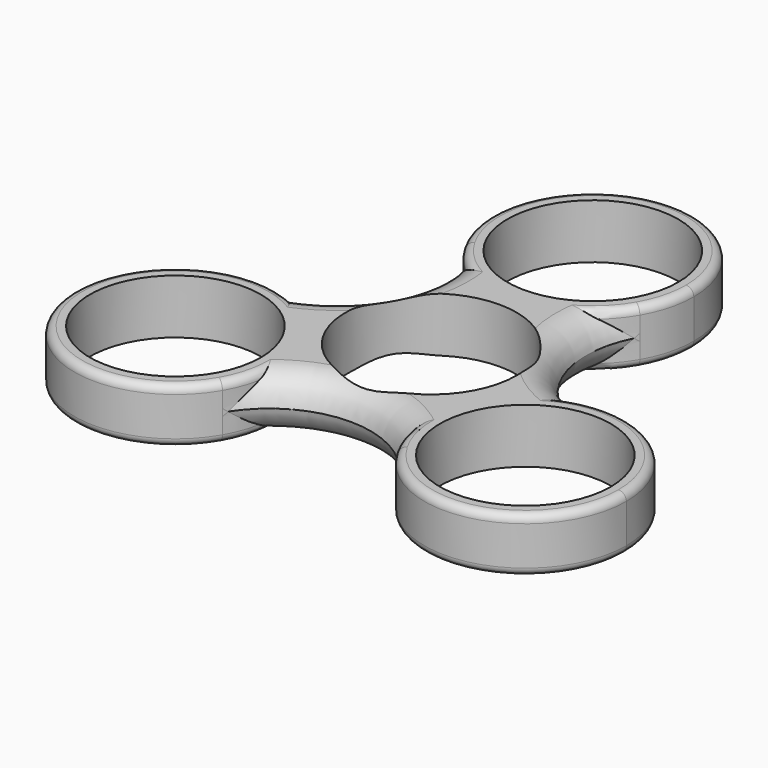
from build123d import *

# Parameters (mm, degrees)
F0_R         = 10.95
F1_DEPTH     = 7
F2_T4_ANGLE  = 119.5195556336
F2_S5_R      = 12.9500003532
F2_T6_DEPTH  = 18
F2_S7_R      = 12.9500003532
F2_T8_DEPTH  = 18
F2_T12_ANGLE = 119.5195556336
F2_S13_R     = 12.9500003532
F2_T14_DEPTH = 21
F2_S15_R     = 12.9500003532
F2_T16_DEPTH = 21
F2_T20_ANGLE = 119.5195556336
F2_S21_R     = 12.9500003532
F2_T22_DEPTH = 22
F2_S23_R     = 12.9500003532
F2_T24_DEPTH = 22
F2_T28_ANGLE = 119.5195556336
F2_S29_R     = 12.9500003532
F2_T30_DEPTH = 18
F2_S31_R     = 12.9500003532
F2_T32_DEPTH = 18
F2_T36_ANGLE = 119.5195556336
F2_S37_R     = 12.9500003532
F2_T38_DEPTH = 21
F2_S39_R     = 12.9500003532
F2_T40_DEPTH = 21
F2_T44_ANGLE = 119.5195556336
F2_S45_R     = 12.9500003532
F2_T46_DEPTH = 22
F2_S47_R     = 12.9500003532
F2_T48_DEPTH = 22
F3_R         = 1
F4_R         = 1


# Not quite as in the source:
# - a fillet or chamfer that OpenCascade refuses, or shapes differently, is made with other operations: its cross-section is extruded or revolved along the edge and cut away or added


with BuildPart() as f1:
    # F0 (on Top) → F1 (new body)
    with BuildSketch(Plane.XY):
        with BuildLine():
            ThreePointArc((-4.7e-08, 12.9500003532), (9.1570330495, 9.1570330827), (12.9500003532, 0))
            ThreePointArc((12.9500003532, 0), (12.508739778, -3.3517067761), (11.2150292324, -6.4750002674))
            ThreePointArc((11.2150292324, -6.4750002674), (15.9550583477, -1.7349710945), (22.4300585697, 0))
            ThreePointArc((22.4300585697, 0), (11.2421440333, 6.4906548839), (11.2150292849, 19.4250005297))
            ThreePointArc((11.2150292849, 19.4250005297), (6.4750001562, 14.6849714097), (-4.7e-08, 12.9500003532))
        make_face()
        with BuildLine():
            ThreePointArc((-11.2150293287, -6.4750001007), (-11.2150292747, 6.4750001942), (-4.7e-08, 12.9500003532))
            ThreePointArc((-4.7e-08, 12.9500003532), (-6.4750001969, 14.6849714332), (-11.2150292849, 19.4250005297))
            ThreePointArc((-11.2150292849, 19.4250005297), (-11.2421440333, 6.4906548839), (-22.4300585697, 0))
            ThreePointArc((-22.4300585697, 0), (-15.9550584311, -1.7349710464), (-11.2150293287, -6.4750001007))
        make_face()
        with BuildLine():
            ThreePointArc((-11.2150292849, 19.4250005297), (-6.4750001969, 14.6849714332), (-4.7e-08, 12.9500003532))
            ThreePointArc((-4.7e-08, 12.9500003532), (6.4750001562, 14.6849714097), (11.2150292849, 19.4250005297))
            ThreePointArc((11.2150292849, 19.4250005297), (12.5087397916, 22.5482939808), (12.9500003532, 25.9000007063))
            ThreePointArc((12.9500003532, 25.9000007063), (-3.3517067255, 38.4087404979), (-11.2150292849, 19.4250005297))
        make_face()
        with Locations((0, 25.9000007063)):
            Circle(F0_R, mode=Mode.SUBTRACT)
        with BuildLine():
            ThreePointArc((11.2150292849, -19.4250005297), (9.4800582165, -12.9500004056), (11.2150292324, -6.4750002674))
            ThreePointArc((11.2150292324, -6.4750002674), (-9.62e-08, -12.9500003532), (-11.2150293287, -6.4750001007))
            ThreePointArc((-11.2150293287, -6.4750001007), (-9.9213187895, -9.5982935854), (-9.4800582165, -12.9500003532))
            ThreePointArc((-9.4800582165, -12.9500003532), (-9.9213187781, -16.3017070786), (-11.2150292849, -19.4250005297))
            ThreePointArc((-11.2150292849, -19.4250005297), (0, -12.9813097678), (11.2150292849, -19.4250005297))
        make_face()
        with BuildLine():
            ThreePointArc((22.4300585697, 0), (15.9550583477, -1.7349710945), (11.2150292324, -6.4750002674))
            ThreePointArc((11.2150292324, -6.4750002674), (9.4800582165, -12.9500004056), (11.2150292849, -19.4250005297))
            ThreePointArc((11.2150292849, -19.4250005297), (25.7817652952, -25.4587401447), (35.3800589229, -12.9500003532))
            ThreePointArc((35.3800589229, -12.9500003532), (31.5870916358, -3.7929672871), (22.4300585697, 0))
        make_face()
        with Locations((22.4300585697, -12.9500003532)):
            Circle(F0_R, mode=Mode.SUBTRACT)
        with BuildLine():
            ThreePointArc((-9.4800582165, -12.9500003532), (-9.9213187895, -9.5982935854), (-11.2150293287, -6.4750001007))
            ThreePointArc((-11.2150293287, -6.4750001007), (-15.9550584311, -1.7349710464), (-22.4300585697, 0))
            ThreePointArc((-22.4300585697, 0), (-33.6450878546, -19.4250005297), (-11.2150292849, -19.4250005297))
            ThreePointArc((-11.2150292849, -19.4250005297), (-9.9213187781, -16.3017070786), (-9.4800582165, -12.9500003532))
        make_face()
        with Locations((-22.4300585697, -12.9500003532)):
            Circle(F0_R, mode=Mode.SUBTRACT)
        with BuildLine():
            ThreePointArc((11.2150292324, -6.4750002674), (12.508739778, -3.3517067761), (12.9500003532, 0))
            ThreePointArc((12.9500003532, 0), (9.1570330495, 9.1570330827), (-4.7e-08, 12.9500003532))
            ThreePointArc((-4.7e-08, 12.9500003532), (-11.2150292747, 6.4750001942), (-11.2150293287, -6.4750001007))
            ThreePointArc((-11.2150293287, -6.4750001007), (-9.62e-08, -12.9500003532), (11.2150292324, -6.4750002674))
        make_face()
        Circle(F0_R, mode=Mode.SUBTRACT)
    extrude(amount=F1_DEPTH)

    # F2: fillet of radius 4 on 6 edges, made by hand


with BuildPart() as f2_tool2:
    # F2_s3 → F2_t4 (revolve)
    with BuildSketch(Plane(origin=(-11.1333905187, 19.4716794138, 0), x_dir=(0, 0, 1), z_dir=(-0.496364659, 0.86811412, 0))):
        with BuildLine():
            ThreePointArc((2.9990343146, -0.094441514), (5.8284271247, 1.0775313612), (7.0004, 3.9069241714))
            Line((7.0004, 3.9069241714), (7.4005365685, 3.9069241714))
            ThreePointArc((7.4005365685, 3.9069241714), (7.4001365685, 1.9064413287), (7.4001365685, -0.094041514))
            Line((7.4001365685, -0.094041514), (7, -0.4941780826))
            ThreePointArc((7, -0.4941780826), (4.9995171573, -0.4941780826), (2.9990343146, -0.4945780826))
            Line((2.9990343146, -0.4945780826), (2.9990343146, -0.094441514))
        make_face()
    revolve(axis=Axis((-22.4844856895, 12.9814238654, 7), (0, 0, -1)), revolution_arc=F2_T4_ANGLE)

    # F2_s5 → F2_t6 (cut, symmetric)
    with BuildSketch(Plane.XY.offset(3.8)):
        with Locations((-22.4300585697, -12.9500003532)):
            Circle(F2_S5_R)
    extrude(amount=F2_T6_DEPTH, both=True, mode=Mode.SUBTRACT)

    # F2_s7 → F2_t8 (cut, symmetric)
    with BuildSketch(Plane.XY.offset(3.8)):
        with Locations((0, 25.9000007063)):
            Circle(F2_S7_R)
    extrude(amount=F2_T8_DEPTH, both=True, mode=Mode.SUBTRACT)


with BuildPart() as f1_1:
    add(f1.part)

    # F2_t1: cut F2_tool2
    add(f2_tool2.part, mode=Mode.SUBTRACT)


with BuildPart() as f2_tool10:
    # F2_s11 → F2_t12 (revolve)
    with BuildSketch(Plane(origin=(22.429664286, -0.0940406875, 0), x_dir=(0, 0, 1), z_dir=(0.9999912108, -0.0041926558, 0))):
        with BuildLine():
            ThreePointArc((2.9990343146, -0.094441514), (5.8284271247, 1.0775313612), (7.0004, 3.9069241714))
            Line((7.0004, 3.9069241714), (7.4005365685, 3.9069241714))
            ThreePointArc((7.4005365685, 3.9069241714), (7.4001365685, 1.9064413287), (7.4001365685, -0.094041514))
            Line((7.4001365685, -0.094041514), (7, -0.4941780826))
            ThreePointArc((7, -0.4941780826), (4.9995171573, -0.4941780826), (2.9990343146, -0.4945780826))
            Line((2.9990343146, -0.4945780826), (2.9990343146, -0.094441514))
        make_face()
    revolve(axis=Axis((22.4844856895, 12.9814238654, 7), (0, 0, -1)), revolution_arc=F2_T12_ANGLE)

    # F2_s13 → F2_t14 (cut, symmetric)
    with BuildSketch(Plane.XY.offset(5.2)):
        with Locations((22.4300585697, -12.9500003532)):
            Circle(F2_S13_R)
    extrude(amount=F2_T14_DEPTH, both=True, mode=Mode.SUBTRACT)

    # F2_s15 → F2_t16 (cut, symmetric)
    with BuildSketch(Plane.XY.offset(5.2)):
        with Locations((0, 25.9000007063)):
            Circle(F2_S15_R)
    extrude(amount=F2_T16_DEPTH, both=True, mode=Mode.SUBTRACT)


with BuildPart() as f1_2:
    add(f1_1.part)

    # F2_t9: cut F2_tool10
    add(f2_tool10.part, mode=Mode.SUBTRACT)


with BuildPart() as f2_tool18:
    # F2_s19 → F2_t20 (revolve)
    with BuildSketch(Plane(origin=(-11.2962737674, -19.3776387263, 0), x_dir=(0, 0, 1), z_dir=(-0.5036265518, -0.8639214642, 0))):
        with BuildLine():
            ThreePointArc((2.9990343146, -0.094441514), (5.8284271247, 1.0775313612), (7.0004, 3.9069241714))
            Line((7.0004, 3.9069241714), (7.4005365685, 3.9069241714))
            ThreePointArc((7.4005365685, 3.9069241714), (7.4001365685, 1.9064413287), (7.4001365685, -0.094041514))
            Line((7.4001365685, -0.094041514), (7, -0.4941780826))
            ThreePointArc((7, -0.4941780826), (4.9995171573, -0.4941780826), (2.9990343146, -0.4945780826))
            Line((2.9990343146, -0.4945780826), (2.9990343146, -0.094441514))
        make_face()
    revolve(axis=Axis((0, -25.9628477308, 7), (0, 0, -1)), revolution_arc=F2_T20_ANGLE)

    # F2_s21 → F2_t22 (cut, symmetric)
    with BuildSketch(Plane.XY.offset(3.8)):
        with Locations((-22.4300585697, -12.9500003532)):
            Circle(F2_S21_R)
    extrude(amount=F2_T22_DEPTH, both=True, mode=Mode.SUBTRACT)

    # F2_s23 → F2_t24 (cut, symmetric)
    with BuildSketch(Plane.XY.offset(3.8)):
        with Locations((22.4300585697, -12.9500003532)):
            Circle(F2_S23_R)
    extrude(amount=F2_T24_DEPTH, both=True, mode=Mode.SUBTRACT)


with BuildPart() as f1_3:
    add(f1_2.part)

    # F2_t17: cut F2_tool18
    add(f2_tool18.part, mode=Mode.SUBTRACT)


with BuildPart() as f2_tool26:
    # F2_s27 → F2_t28 (revolve)
    with BuildSketch(Plane(origin=(-11.1333905187, 19.4716794138, 0), x_dir=(0, 0, 1), z_dir=(-0.496364659, 0.86811412, 0))):
        with BuildLine():
            ThreePointArc((4.0009656854, -0.094441514), (1.1715728753, 1.0775313612), (-0.0004, 3.9069241714))
            Line((-0.0004, 3.9069241714), (-0.4005365685, 3.9069241714))
            ThreePointArc((-0.4005365685, 3.9069241714), (-0.4001365685, 1.9064413287), (-0.4001365685, -0.094041514))
            Line((-0.4001365685, -0.094041514), (0, -0.4941780826))
            ThreePointArc((0, -0.4941780826), (2.0004828427, -0.4941780826), (4.0009656854, -0.4945780826))
            Line((4.0009656854, -0.4945780826), (4.0009656854, -0.094441514))
        make_face()
    revolve(axis=Axis((-22.4844856895, 12.9814238654, 0), (0, 0, -1)), revolution_arc=F2_T28_ANGLE)

    # F2_s29 → F2_t30 (cut, symmetric)
    with BuildSketch(Plane.XY.offset(3.2)):
        with Locations((-22.4300585697, -12.9500003532)):
            Circle(F2_S29_R)
    extrude(amount=F2_T30_DEPTH, both=True, mode=Mode.SUBTRACT)

    # F2_s31 → F2_t32 (cut, symmetric)
    with BuildSketch(Plane.XY.offset(3.2)):
        with Locations((0, 25.9000007063)):
            Circle(F2_S31_R)
    extrude(amount=F2_T32_DEPTH, both=True, mode=Mode.SUBTRACT)


with BuildPart() as f1_4:
    add(f1_3.part)

    # F2_t25: cut F2_tool26
    add(f2_tool26.part, mode=Mode.SUBTRACT)


with BuildPart() as f2_tool34:
    # F2_s35 → F2_t36 (revolve)
    with BuildSketch(Plane(origin=(22.429664286, -0.0940406875, 0), x_dir=(0, 0, 1), z_dir=(0.9999912108, -0.0041926558, 0))):
        with BuildLine():
            ThreePointArc((4.0009656854, -0.094441514), (1.1715728753, 1.0775313612), (-0.0004, 3.9069241714))
            Line((-0.0004, 3.9069241714), (-0.4005365685, 3.9069241714))
            ThreePointArc((-0.4005365685, 3.9069241714), (-0.4001365685, 1.9064413287), (-0.4001365685, -0.094041514))
            Line((-0.4001365685, -0.094041514), (0, -0.4941780826))
            ThreePointArc((0, -0.4941780826), (2.0004828427, -0.4941780826), (4.0009656854, -0.4945780826))
            Line((4.0009656854, -0.4945780826), (4.0009656854, -0.094441514))
        make_face()
    revolve(axis=Axis((22.4844856895, 12.9814238654, 0), (0, 0, -1)), revolution_arc=F2_T36_ANGLE)

    # F2_s37 → F2_t38 (cut, symmetric)
    with BuildSketch(Plane.XY.offset(1.8)):
        with Locations((22.4300585697, -12.9500003532)):
            Circle(F2_S37_R)
    extrude(amount=F2_T38_DEPTH, both=True, mode=Mode.SUBTRACT)

    # F2_s39 → F2_t40 (cut, symmetric)
    with BuildSketch(Plane.XY.offset(1.8)):
        with Locations((0, 25.9000007063)):
            Circle(F2_S39_R)
    extrude(amount=F2_T40_DEPTH, both=True, mode=Mode.SUBTRACT)


with BuildPart() as f1_5:
    add(f1_4.part)

    # F2_t33: cut F2_tool34
    add(f2_tool34.part, mode=Mode.SUBTRACT)


with BuildPart() as f2_tool42:
    # F2_s43 → F2_t44 (revolve)
    with BuildSketch(Plane(origin=(-11.2962737674, -19.3776387263, 0), x_dir=(0, 0, 1), z_dir=(-0.5036265518, -0.8639214642, 0))):
        with BuildLine():
            ThreePointArc((4.0009656854, -0.094441514), (1.1715728753, 1.0775313612), (-0.0004, 3.9069241714))
            Line((-0.0004, 3.9069241714), (-0.4005365685, 3.9069241714))
            ThreePointArc((-0.4005365685, 3.9069241714), (-0.4001365685, 1.9064413287), (-0.4001365685, -0.094041514))
            Line((-0.4001365685, -0.094041514), (0, -0.4941780826))
            ThreePointArc((0, -0.4941780826), (2.0004828427, -0.4941780826), (4.0009656854, -0.4945780826))
            Line((4.0009656854, -0.4945780826), (4.0009656854, -0.094441514))
        make_face()
    revolve(axis=Axis((0, -25.9628477308, 0), (0, 0, -1)), revolution_arc=F2_T44_ANGLE)

    # F2_s45 → F2_t46 (cut, symmetric)
    with BuildSketch(Plane.XY.offset(3.2)):
        with Locations((-22.4300585697, -12.9500003532)):
            Circle(F2_S45_R)
    extrude(amount=F2_T46_DEPTH, both=True, mode=Mode.SUBTRACT)

    # F2_s47 → F2_t48 (cut, symmetric)
    with BuildSketch(Plane.XY.offset(3.2)):
        with Locations((22.4300585697, -12.9500003532)):
            Circle(F2_S47_R)
    extrude(amount=F2_T48_DEPTH, both=True, mode=Mode.SUBTRACT)


with BuildPart() as f1_6:
    add(f1_5.part)

    # F2_t41: cut F2_tool42
    add(f2_tool42.part, mode=Mode.SUBTRACT)

    # F3
    f3_edges = [f1_6.edges().sort_by_distance(p)[0] for p in [
        (0, 38.850001, 7),
        (9.80296, -15.823828, 7),
        (-33.645088, -19.425001, 7),
    ]]
    fillet(f3_edges, radius=F3_R)

    # F4
    f4_edges = [f1_6.edges().sort_by_distance(p)[0] for p in [
        (0, 38.850001, 0),
        (-33.645088, -19.425001, 0),
        (9.80296, -15.823828, 0),
        (-18.605317, -0.577698, 0),
        (-9.80296, -15.823829, 0),
        (-8.802357, 16.401526, 0),
        (8.802357, 16.401526, 0),
        (18.605317, -0.577698, 0),
        (33.645088, -19.425001, 0),
    ]]
    fillet(f4_edges, radius=F4_R)


solid = f1_6.part
